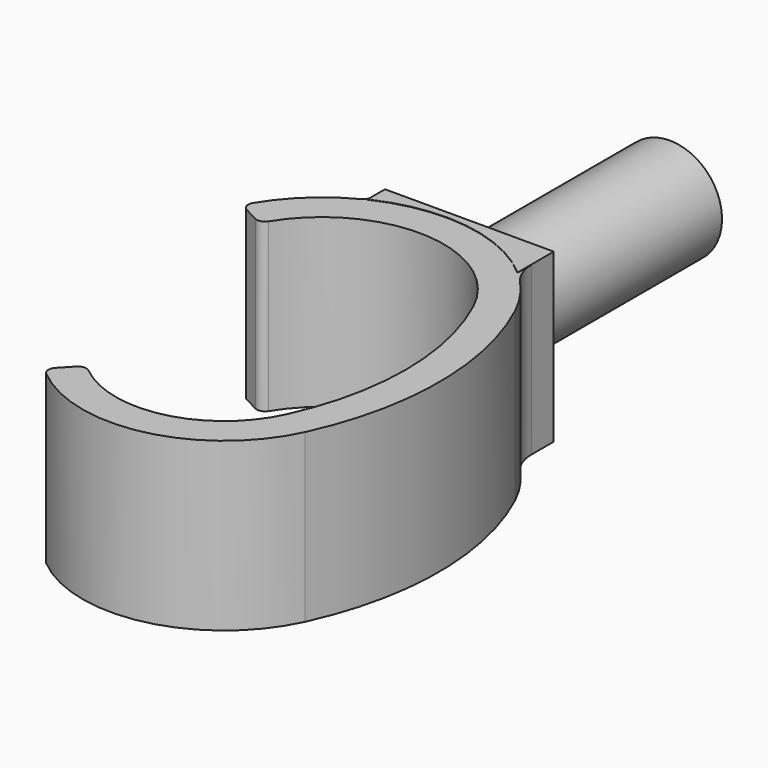
from build123d import *

# Parameters (mm, degrees)
F1_DEPTH      = 20
F4_END_RADIUS = 18.58687693
F3_W          = 20.205357112
F3_H          = 20.0386047363
F4_REACH      = 81.284821593
F5_R          = 1
F6_R          = 5
F7_R          = 1
F8_R          = 6.25
F9_DEPTH      = 30


# Not quite as in the source:
# - a feature of the source that left no trace in its solid (it failed there, or was rolled back) is left out


with BuildPart() as f1:
    # F0 (on Top) → F1 (new body)
    with BuildSketch(Plane.XY):
        with BuildLine():
            ThreePointArc((-16.300464081, 12.3786436003), (-3.0365664125, 20.1688822052), (9.8326279785, 11.7425760982))
            ThreePointArc((9.8326279785, 11.7425760982), (12.939174946, -2.2913182786), (9.8326279785, -16.3252126554))
            ThreePointArc((9.8326279785, -16.3252126554), (0.5036385974, -23.5957971339), (-10.8497184243, -20.2802691412))
            Line((-10.8497184243, -20.2802691412), (-13.5972941331, -23.1872998815))
            ThreePointArc((-13.5972941331, -23.1872998815), (1.2549394728, -27.5246070039), (13.4589359939, -18.0133744302))
            ThreePointArc((13.4589359939, -18.0133744302), (16.939174946, -2.2913182786), (13.4589359939, 13.430737873))
            ThreePointArc((13.4589359939, 13.430737873), (-2.9392370682, 24.1676979047), (-19.8403485782, 14.2412272216))
            Line((-19.8403485782, 14.2412272216), (-16.300464081, 12.3786436003))
        make_face()
    extrude(amount=F1_DEPTH)

    f4_end = (Plane(origin=(-3.391499204, 5.5863240865, 10), x_dir=(-1, 0, 0), z_dir=(0, 0, -1)) * Cylinder(F4_END_RADIUS, 296.0871828679, mode=Mode.PRIVATE)).faces().sort_by_distance((-2.9392370682, 24.1676979047, 10))[0]
    # F3 (on offset) → F4 (join, up to the whole of a round face its end follows)
    with BuildSketch(Plane.XZ.offset(-25)):
        with Locations((-1.2632482685, 10.0193023682)):
            Rectangle(F3_W, F3_H)
    f4_long = extrude(amount=F4_REACH, mode=Mode.PRIVATE)
    add(split(f4_long, bisect_by=f4_end, keep=Keep.ALL, mode=Mode.PRIVATE).solids().sort_by_distance((-1.2632482685, 25, 10.0193023682))[0])

    # F5
    f5_edges = [f1.edges().sort_by_distance(p)[0] for p in [
        (-16.300464, 12.378644, 10),
        (-19.840349, 14.241227, 10),
        (-10.849718, -20.280269, 10),
        (-13.597294, -23.1873, 10),
    ]]
    fillet(f5_edges, radius=F5_R)

    # F6
    f6_edges = [f1.edges().sort_by_distance(p)[0] for p in [
        (8.83943, 19.581908, 10),
    ]]
    fillet(f6_edges, radius=F6_R)

    # F7
    f7_edges = [f1.edges().sort_by_distance(p)[0] for p in [
        (-11.365927, 22.375621, 10),
    ]]
    fillet(f7_edges, radius=F7_R)

    # F8 (on face) → F9 (join)
    with BuildSketch(Plane(origin=(0, 25, 0), x_dir=(-1, 0, 0), z_dir=(0, 1, 0))):
        with Locations((1.2632482685, 10.0193023682)):
            Circle(F8_R)
    extrude(amount=F9_DEPTH)


solid = f1.part
